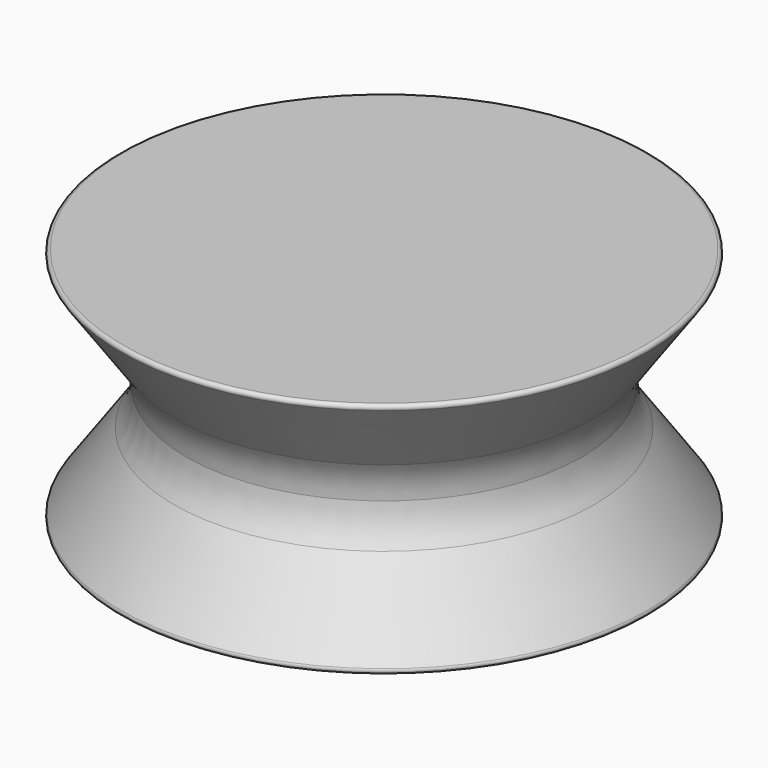
from build123d import *
from build123d import SkipClean  # not in build123d's __all__


# Not quite as in the source:
# - ends of sketch curves that miss each other by under 0.0002 mm in the source are joined


with BuildPart() as f1:
    # F0 (on Front) → F1 (revolve)
    with BuildSketch(Plane.XZ):
        with BuildLine():
            ThreePointArc((150, 0), (152.3425507406, 15.1250629778), (159.1507012033, 28.8328768565))
            Line((159.1507012033, 28.8328768565), (199.542465, 86.058356))
            ThreePointArc((199.542465, 86.058356), (199.7196970287, 88.6501935058), (197.5, 90))
            Line((197.5, 90), (0, 90))
            Line((0, 90), (0, 0))
            Line((0, 0), (150, 0))
        make_face()
    revolve(axis=Axis((0, 0, 45), (0, 0, 1)))

    # F2: F1 across face


with BuildPart() as f1_1:
    add(f1.part, clean=False)
    with SkipClean():  # cleaning this boolean's faces spoils the solid; the shape is the same uncleaned
        add(f1.part.mirror(Plane(origin=(0, 0, 0), x_dir=(1, 0, 0), z_dir=(0, 0, -1))), clean=False)


solid = f1_1.part
